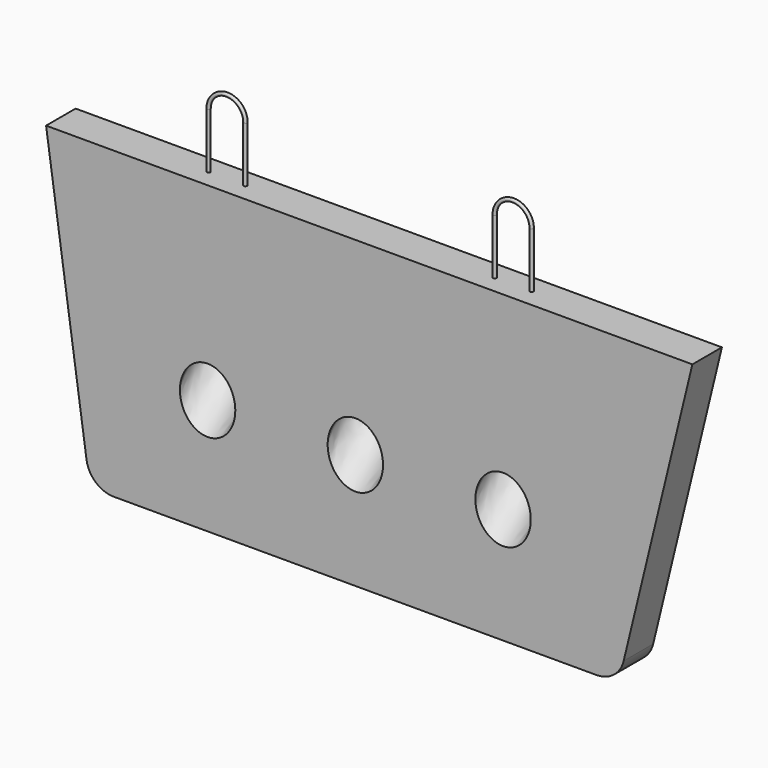
from build123d import *

# Parameters (mm, degrees)
F1_DEPTH = 50.8
F5_R     = 2.38125
F8_W     = 889
F8_H     = 50.8
F8_R     = 2.38125
F9_DEPTH = 0.00254


# Not quite as in the source:
# - a pattern or mirror of a feature is missing from the dataset's text; its kind, count and spacing are read off the source's solid


with BuildPart() as f1:
    # F0 (on Front) → F1 (new body)
    with BuildSketch(Plane.XZ):
        with BuildLine():
            Line((-425.3831805585, 419.1), (-369.7609472035, 32.6718524805))
            ThreePointArc((-369.7609472035, 32.6718524805), (-356.9975280935, 9.3039723183), (-332.0496065417, 0))
            Line((-332.0496065417, 0), (332.0496065417, 0))
            ThreePointArc((332.0496065417, 0), (355.6039123775, 8.1533027431), (369.0770955684, 29.1236390238))
            Line((369.0770955684, 29.1236390238), (463.6168194415, 419.1))
            Line((463.6168194415, 419.1), (-425.3831805585, 419.1))
        make_face()
    extrude(amount=F1_DEPTH)

    # F4: sweep along a path in F3
    with BuildLine(Plane.YZ) as f4_path:
        Line((-50.8, 158.75), (0, 203.2))
    # F2 (on face) → F4 (sweep, cut)
    with BuildSketch(Plane.XZ.offset(50.8)):
        with BuildLine():
            add(Edge.make_bspline(
                [(-203.2039687112, 114.3), (-137.2128329429, 114.3), (-170.2084008271, 180.975), (-203.2039687112, 247.65), (-236.1995365954, 180.975), (-269.1951044796, 114.3), (-203.2039687112, 114.3)],
                knots=[0, 0, 0, 2.0943951024, 2.0943951024, 4.1887902048, 4.1887902048, 6.2831853072, 6.2831853072, 6.2831853072], degree=2, weights=[1, 0.5, 1, 0.5, 1, 0.5, 1]))
        make_face()
        with BuildLine():
            add(Edge.make_bspline(
                [(0, 114.3), (65.9911357684, 114.3), (32.9955678842, 180.975), (0, 247.65), (-32.9955678842, 180.975), (-65.9911357684, 114.3), (0, 114.3)],
                knots=[0, 0, 0, 2.0943951024, 2.0943951024, 4.1887902048, 4.1887902048, 6.2831853072, 6.2831853072, 6.2831853072], degree=2, weights=[1, 0.5, 1, 0.5, 1, 0.5, 1]))
        make_face()
        with BuildLine():
            add(Edge.make_bspline(
                [(203.2039687112, 114.3), (269.1951044796, 114.3), (236.1995365954, 180.975), (203.2039687112, 247.65), (170.2084008271, 180.975), (137.2128329429, 114.3), (203.2039687112, 114.3)],
                knots=[0, 0, 0, 2.0943951024, 2.0943951024, 4.1887902048, 4.1887902048, 6.2831853072, 6.2831853072, 6.2831853072], degree=2, weights=[1, 0.5, 1, 0.5, 1, 0.5, 1]))
        make_face()
    sweep(path=f4_path.line, mode=Mode.SUBTRACT)

    # F7: sweep along a path in F6
    with BuildLine(Plane.XZ) as f7_path:
        Line((-222.25, 419.1), (-222.25, 495.3))
        ThreePointArc((-222.25, 495.3), (-196.85, 520.7), (-171.45, 495.3))
        Line((-171.45, 495.3), (-171.45, 419.1))
    # F5 (on face) → F7 (sweep)
    with BuildSketch(Plane.XY.offset(419.1)):
        with Locations((-222.25, -25.4)):
            Circle(F5_R)
    f7 = sweep(path=f7_path.line)

    # F7_copies: F7 across plane
    add(f7.mirror(Plane(origin=(0, 0, 0), x_dir=(0, 0, 1), z_dir=(1, 0, 0))))


with BuildPart() as f9:
    # F8 (on face) → F9 (new body)
    with BuildSketch(Plane.XY.offset(419.1)):
        with Locations((19.1168194415, -25.4)):
            Rectangle(F8_W, F8_H)
        with Locations((-222.25, -25.4)):
            Circle(F8_R, mode=Mode.SUBTRACT)
        with Locations((-171.45, -25.4)):
            Circle(F8_R, mode=Mode.SUBTRACT)
        with Locations((171.45, -25.4)):
            Circle(F8_R, mode=Mode.SUBTRACT)
        with Locations((222.25, -25.4)):
            Circle(F8_R, mode=Mode.SUBTRACT)
    extrude(amount=F9_DEPTH)


solid = Compound([f1.part, f9.part])
